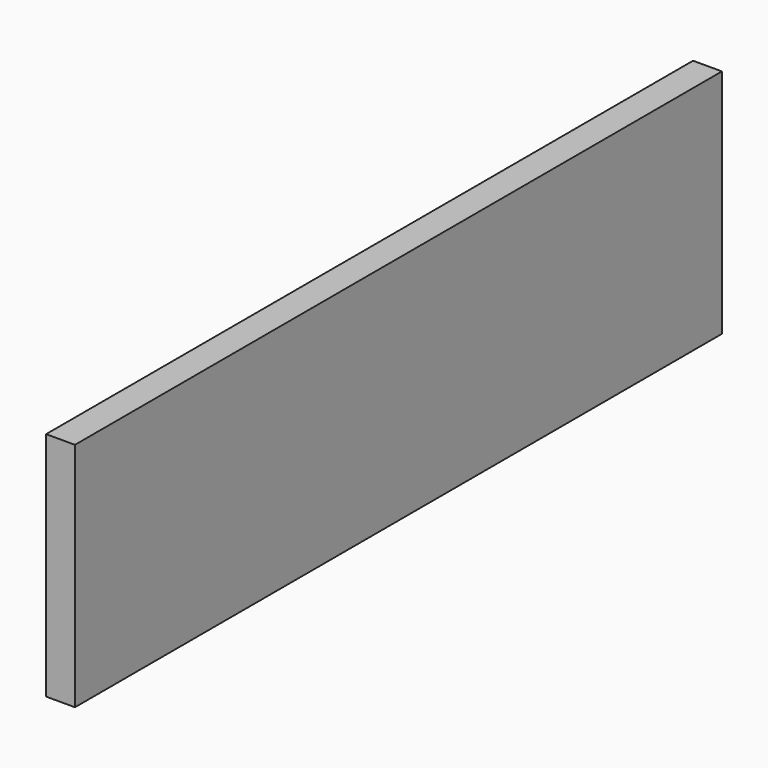
from build123d import *

# Parameters (mm, degrees)
F2_W     = 3.175
F2_H     = 25.4
F3_DEPTH = 88.9


# Not quite as in the source:
# - a feature of the source that left no trace in its solid (it failed there, or was rolled back) is left out


with BuildPart() as f3:
    # F2 (on Front) → F3 (new body)
    with BuildSketch(Plane.XZ):
        with Locations((-46.4678156614, 15.1370579049)):
            Rectangle(F2_W, F2_H)
    extrude(amount=-F3_DEPTH)


solid = f3.part
